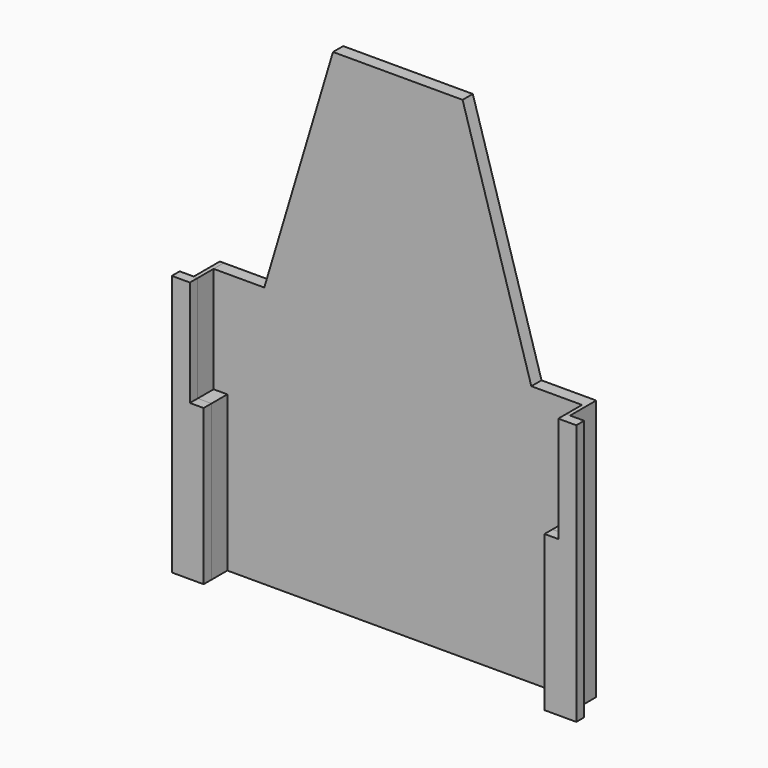
from build123d import *

# Parameters (mm, degrees)
F0_W     = 3.5839973688
F0_H     = 66.5
F1_DEPTH = 2.5
F2_DEPTH = 8.3
F4_DEPTH = 3.25


with BuildPart() as f1:
    # F0 (on Front) → F1 (new body)
    with BuildSketch(Plane.XZ):
        with Locations((-24.1530238986, -11.5398805141)):
            Rectangle(F0_W, F0_H)
        Polygon((-21.345022583, 21.7101194859), (-22.3610252142, 21.7101194859), (-22.3610252142, -44.7898805141), (-17.845022583, -44.7898805141), (-17.845022583, -5.2898805141), (-21.345022583, -5.2898805141), align=None)
    extrude(amount=F1_DEPTH)


with BuildPart() as f1b:
    # F0 (on Front) → F1, piece 2 (new body)
    with BuildSketch(Plane.XZ):
        with Locations((75.2629787326, -11.5398805141)):
            Rectangle(F0_W, F0_H)
        Polygon((68.954977417, -5.2898805141), (68.954977417, -44.7898805141), (73.4709800482, -44.7898805141), (73.4709800482, 21.7101194859), (72.454977417, 21.7101194859), (72.454977417, -5.2898805141), align=None)
    extrude(amount=F1_DEPTH)


with BuildPart() as f2:
    # F0 (on Front) → F2 (new body)
    with BuildSketch(Plane.XZ):
        Polygon((-21.345022583, 21.7101194859), (-22.3610252142, 21.7101194859), (-22.3610252142, -44.7898805141), (-17.845022583, -44.7898805141), (-17.845022583, -5.2898805141), (-21.345022583, -5.2898805141), align=None)
    extrude(amount=-F2_DEPTH)


with BuildPart() as f2b:
    # F0 (on Front) → F2, piece 2 (new body)
    with BuildSketch(Plane.XZ):
        Polygon((68.954977417, -5.2898805141), (68.954977417, -44.7898805141), (73.4709800482, -44.7898805141), (73.4709800482, 21.7101194859), (72.454977417, 21.7101194859), (72.454977417, -5.2898805141), align=None)
    extrude(amount=-F2_DEPTH)

    # F3 (on face) → F4 (join)
    with BuildSketch(Plane(origin=(0, 8.3, 0), x_dir=(-1, 0, 0), z_dir=(0, 1, 0))):
        Polygon((21.345022583, -5.2898805141), (21.345022583, 21.7101194859), (8.4450252142, 21.7101194859), (-25.5549747858, 21.7101194859), (-25.5549747858, -44.7898805141), (17.845022583, -44.7898805141), (17.845022583, -5.2898805141), align=None)
        Polygon((-25.5549747858, 21.7101194859), (8.4450252142, 21.7101194859), (-9.0549747858, 80.2101194859), (-25.5549747858, 80.2101194859), align=None)
        Polygon((-59.5549747858, 21.7101194859), (-25.5549747858, 21.7101194859), (-25.5549747858, 80.2101194859), (-42.0549747858, 80.2101194859), align=None)
        Polygon((-73.4709747858, -44.7898805141), (-25.5549747858, -44.7898805141), (-25.5549747858, 21.7101194859), (-59.5549747858, 21.7101194859), (-73.4709747858, 21.7101194859), align=None)
    extrude(amount=-F4_DEPTH)


solid = Compound([f1.part, f1b.part, f2.part, f2b.part])
